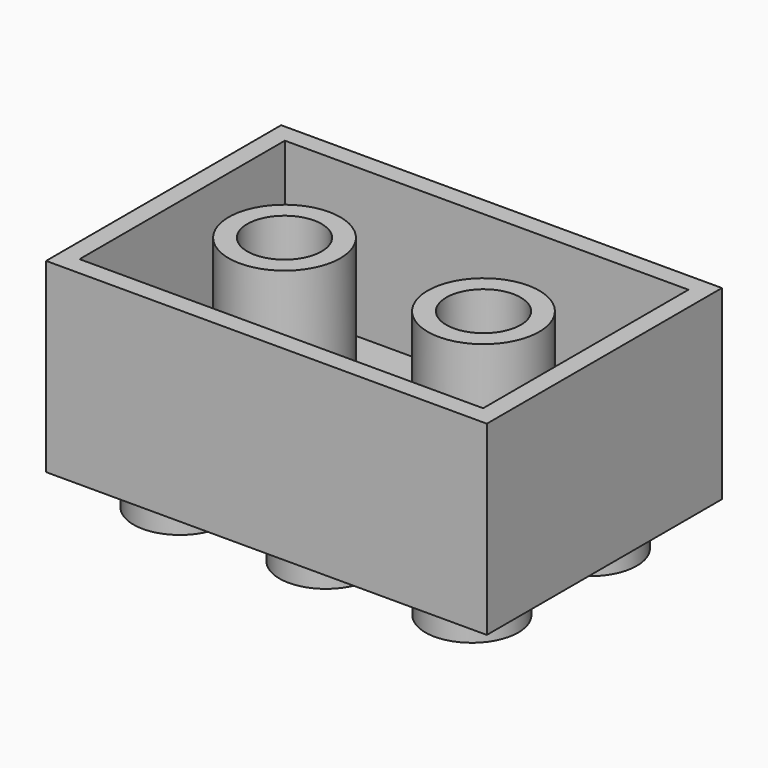
from build123d import *

# Parameters (mm, degrees)
F0_W      = 23.7
F0_H      = 15.8
F1_DEPTH  = 10
F9_W      = 21.7
F9_H      = 13.8
F10_DEPTH = 8
F11_R     = 3
F11_R_2   = 2
F12_DEPTH = 8
F15_R     = 2.5
F16_DEPTH = 2


# Not quite as in the source:
# - the program builds the solid bodies; features that only make, move or delete a surface that nothing else refers to are left out


with BuildPart() as f1:
    # F0 (on Top) → F1 (new body)
    with BuildSketch(Plane.XY):
        Rectangle(F0_W, F0_H)
    extrude(amount=F1_DEPTH)

    # F9 (on face) → F10 (cut)
    with BuildSketch(Plane.XY.offset(10)):
        Rectangle(F9_W, F9_H)
    extrude(amount=-F10_DEPTH, mode=Mode.SUBTRACT)

    # F11 (on face) → F12 (join, through all)
    with BuildSketch(Plane.XY.offset(2)):
        with Locations((-5.35, 0)):
            Circle(F11_R)
        with Locations((-5.35, 0)):
            Circle(F11_R_2, mode=Mode.SUBTRACT)
    extrude(amount=F12_DEPTH)

    # F13: F1 across plane


with BuildPart() as f1_1:
    add(f1.part)
    add(f1.part.mirror(Plane.YZ))


with BuildPart() as f16:
    # F15 (on face) → F16 (new body)
    with BuildSketch(Plane(origin=(0, 0, 0), x_dir=(1, 0, 0), z_dir=(0, 0, -1))):
        with Locations((-7.752910628, -3.9399788514)):
            Circle(F15_R)
    extrude(amount=F16_DEPTH)


with BuildPart() as f16b:
    # F15 (on face) → F16, piece 2 (new body)
    with BuildSketch(Plane(origin=(0, 0, 0), x_dir=(1, 0, 0), z_dir=(0, 0, -1))):
        with Locations((-7.85, 3.9)):
            Circle(F15_R)
    extrude(amount=F16_DEPTH)


with BuildPart() as f16c:
    # F15 (on face) → F16, piece 3 (new body)
    with BuildSketch(Plane(origin=(0, 0, 0), x_dir=(1, 0, 0), z_dir=(0, 0, -1))):
        with Locations((-0.00219, 3.9)):
            Circle(F15_R)
    extrude(amount=F16_DEPTH)


with BuildPart() as f16d:
    # F15 (on face) → F16, piece 4 (new body)
    with BuildSketch(Plane(origin=(0, 0, 0), x_dir=(1, 0, 0), z_dir=(0, 0, -1))):
        with Locations((7.84562, 3.9)):
            Circle(F15_R)
    extrude(amount=F16_DEPTH)


with BuildPart() as f16e:
    # F15 (on face) → F16, piece 5 (new body)
    with BuildSketch(Plane(origin=(0, 0, 0), x_dir=(1, 0, 0), z_dir=(0, 0, -1))):
        with Locations((7.942709372, -3.9399788514)):
            Circle(F15_R)
    extrude(amount=F16_DEPTH)


with BuildPart() as f16f:
    # F15 (on face) → F16, piece 6 (new body)
    with BuildSketch(Plane(origin=(0, 0, 0), x_dir=(1, 0, 0), z_dir=(0, 0, -1))):
        with Locations((0.094899372, -3.9399788514)):
            Circle(F15_R)
    extrude(amount=F16_DEPTH)


solid = Compound([f1_1.part, f16.part, f16b.part, f16c.part, f16d.part, f16e.part, f16f.part])
